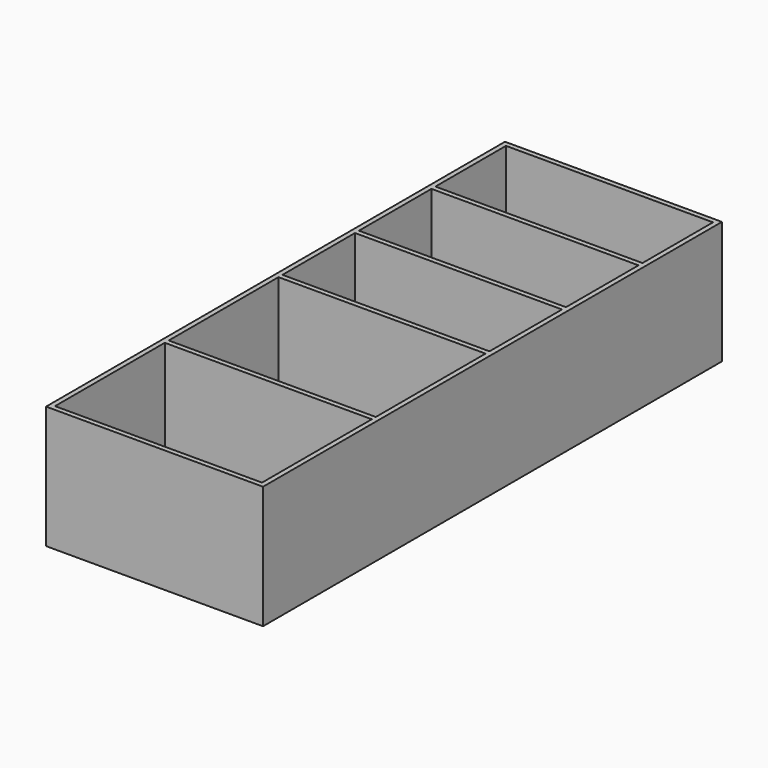
from build123d import *

# Parameters (mm, degrees)
F0_W     = 43.8
F0_H     = 115.8
F1_DEPTH = 1
F2_W     = 41.8
F2_H     = 1
F3_DEPTH = 23.8


# Not quite as in the source:
# - a feature names something its author has since deleted; it is built from what else it names


with BuildPart() as f1:
    # F0 (on Top) → F1 (new body)
    with BuildSketch(Plane.XY):
        with Locations((21.9, -57.9)):
            Rectangle(F0_W, F0_H)
    extrude(amount=F1_DEPTH)

    # F2 (on face) → F3 (join)
    with BuildSketch(Plane.XY.offset(1)):
        Polygon((0, -114.8), (0, -115.8), (43.8, -115.8), (43.8, -114.8), (42.8, -114.8), (1, -114.8), align=None)
        Polygon((0, 0), (0, -114.8), (1, -114.8), (1, -87.35), (1, -87.1), (1, -86.35), (1, -86.1), (1, -58.4), (1, -57.4), (1, -39.1), (1, -38.1), (1, -19.8), (1, -18.8), (1, -1), (1, 0), align=None)
        Polygon((42.8, -114.8), (43.8, -114.8), (43.8, 0), (42.8, 0), (42.8, -1), (42.8, -18.8), (42.8, -19.8), (42.8, -38.1), (42.8, -39.1), (42.8, -57.4), (42.8, -58.4), (42.8, -86.1), (42.8, -87.1), align=None)
        with Locations((21.9, -0.5)):
            Rectangle(F2_W, F2_H)
        with Locations((21.9, -19.3)):
            Rectangle(F2_W, F2_H)
        with Locations((21.9, -38.6)):
            Rectangle(F2_W, F2_H)
        with Locations((21.9, -57.9)):
            Rectangle(F2_W, F2_H)
        Polygon((1, -87.1), (42.8, -87.1), (42.8, -86.1), (1, -86.1), (1, -86.35), align=None)
    extrude(amount=F3_DEPTH)


solid = f1.part
